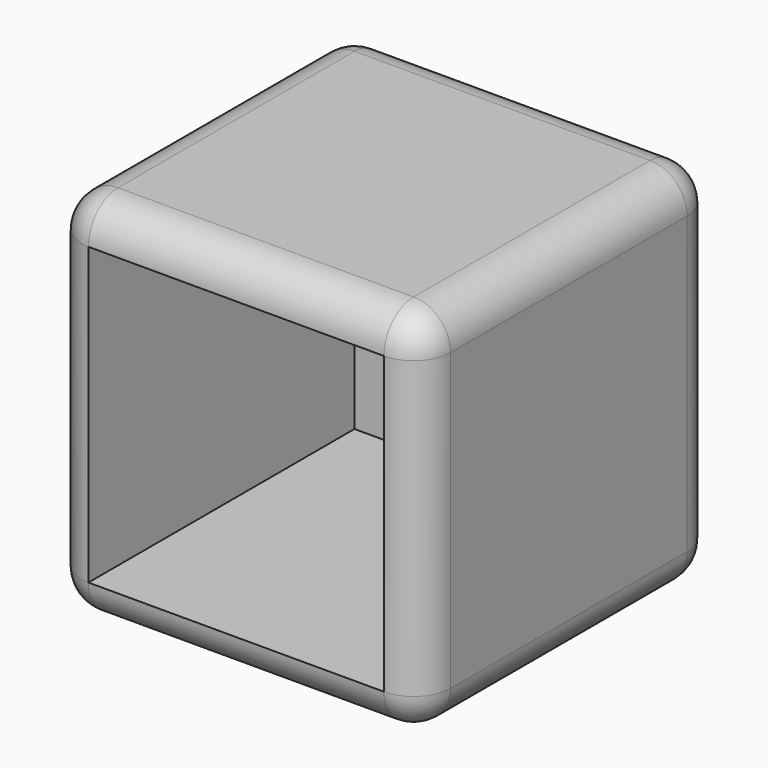
from build123d import *

# Parameters (mm, degrees)
F0_W     = 25
F0_H     = 25
F1_DEPTH = 25
F2_T     = -2.5
F3_R     = 2.49999


# Not quite as in the source:
# - a fillet or chamfer is up to 0.001 mm smaller than in the source, because OpenCascade refuses the exact size


with BuildPart() as f1:
    # F0 (on Top) → F1 (new body)
    with BuildSketch(Plane.XY):
        with Locations((12.5, 12.5)):
            Rectangle(F0_W, F0_H)
    extrude(amount=F1_DEPTH)

    # F2
    f2_openings = [f1.faces().sort_by_distance(p)[0] for p in [
        (12.5, 0, 12.5),
    ]]
    offset(amount=F2_T, openings=f2_openings)

    # F3 (radius 2.5 in the source; OpenCascade refuses exactly that, so slightly less here)
    f3_edges = [f1.edges().sort_by_distance(p)[0] for p in [
        (12.5, 0, 25),
        (25, 12.5, 0),
        (12.5, 25, 0),
        (0, 12.5, 0),
        (25, 12.5, 25),
        (12.5, 25, 25),
        (0, 25, 12.5),
        (0, 0, 12.5),
        (0, 12.5, 25),
        (25, 0, 12.5),
        (25, 25, 12.5),
        (12.5, 0, 0),
    ]]
    fillet(f3_edges, radius=F3_R)


solid = f1.part
